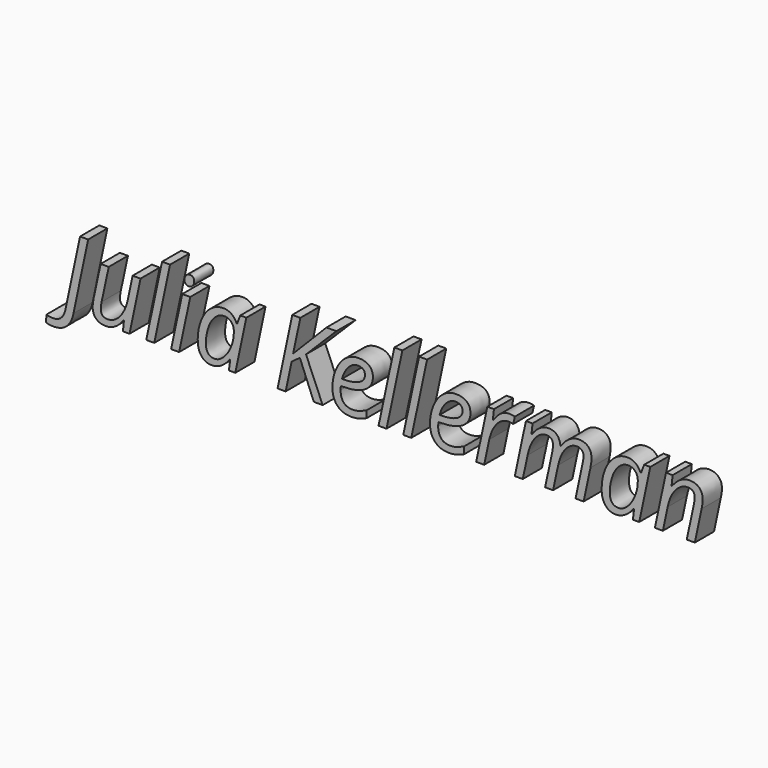
from build123d import *

# Parameters (mm, degrees)
F0_TEXT_SIZE = 154.6762831923
F1_DEPTH     = 38.1


# Not quite as in the source:
# - Text() gives the source's letters only with a copy of the font that has no kerning and outlines rounded to 1/6400 em; it was checked with that copy


with BuildPart() as f1:
    # F0 (on Front) → F1 (new body)
    with BuildSketch(Plane.XZ):
        with Locations((-1817.920807749, -345.3132222639)):
            Text('Julia Kellerman', F0_TEXT_SIZE, font='Open Sans', font_style=FontStyle.ITALIC, text_align=(TextAlign.LEFT, TextAlign.BOTTOM))
    extrude(amount=F1_DEPTH)


solid = f1.part
